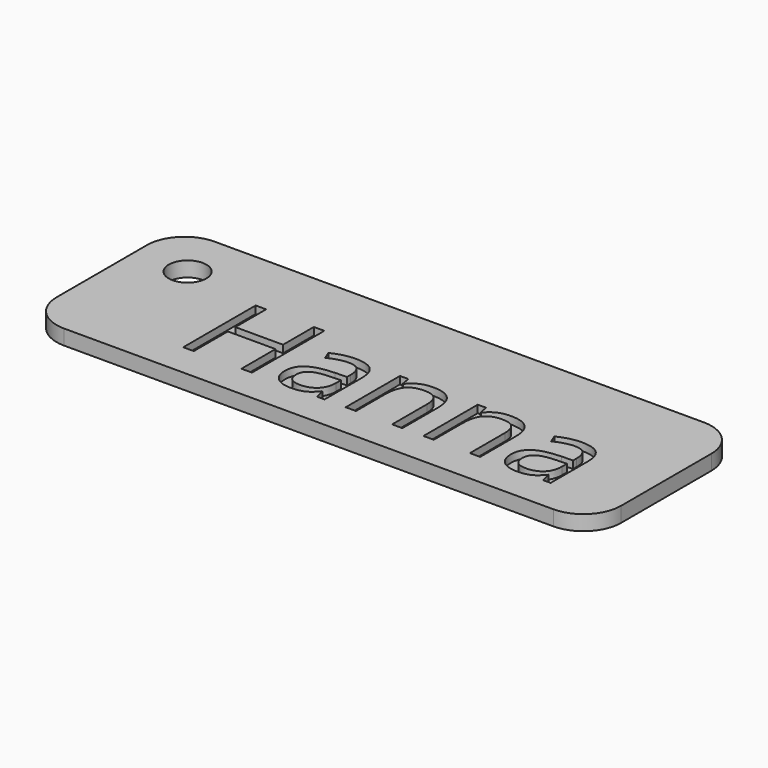
from build123d import *

# Parameters (mm, degrees)
F1_DEPTH     = 2
F3_D         = 5
F4_TEXT_SIZE = 16.8377714646
F5_DEPTH     = 1


# Not quite as in the source:
# - Text() gives the source's letters only with a copy of the font that has no kerning and outlines rounded to 1/6400 em; it was checked with that copy


with BuildPart() as f1:
    # F0 (on Top) → F1 (new body)
    with BuildSketch(Plane.XY):
        with BuildLine():
            ThreePointArc((-37.5, -7.5), (-36.0355339059, -11.0355339059), (-32.5, -12.5))
            Line((-32.5, -12.5), (32.5, -12.5))
            ThreePointArc((32.5, -12.5), (36.0355339059, -11.0355339059), (37.5, -7.5))
            Line((37.5, -7.5), (37.5, 7.5))
            ThreePointArc((37.5, 7.5), (36.0355339059, 11.0355339059), (32.5, 12.5))
            Line((32.5, 12.5), (-32.5, 12.5))
            ThreePointArc((-32.5, 12.5), (-36.0355339059, 11.0355339059), (-37.5, 7.5))
            Line((-37.5, 7.5), (-37.5, -7.5))
        make_face()
    extrude(amount=F1_DEPTH)

    # F3 (through all)
    with Locations(Plane.XY.offset(2)):
        with Locations((-30.5, 5.5)):
            Hole(F3_D / 2)

    # F4 (on face) → F5 (cut)
    with BuildSketch(Plane.XY.offset(2)):
        with Locations((-21.8750014901, -8.0586364493)):
            Text('Hanna', F4_TEXT_SIZE, font='Open Sans', text_align=(TextAlign.LEFT, TextAlign.BOTTOM))
    extrude(amount=-F5_DEPTH, mode=Mode.SUBTRACT)


solid = f1.part
